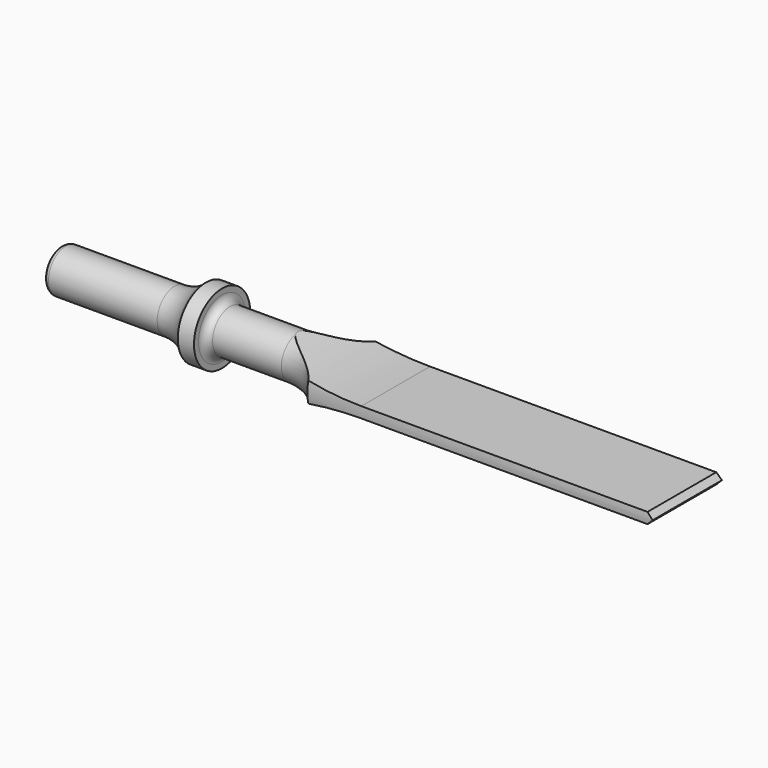
from build123d import *

# Parameters (mm, degrees)
F3_DEPTH = 25.4
F4_DEPTH = 25.4


# Not quite as in the source:
# - ends of sketch curves that miss each other by under 0.0002 mm in the source are joined


with BuildPart() as f1:
    # F0 (on Front) → F1 (revolve)
    with BuildSketch(Plane.XZ):
        with BuildLine():
            Line((0, 4.826), (0, 0))
            Line((0, 0), (184.15, 0))
            Line((184.15, 0), (184.15, 12.7))
            Line((184.15, 12.7), (82.55, 12.7))
            ThreePointArc((82.55, 12.7), (76.9495160289, 8.0259690987), (69.8500007868, 6.350001049))
            Line((69.8500007868, 6.350001049), (49.657, 6.35))
            ThreePointArc((49.657, 6.35), (48.0405538982, 7.0195538982), (47.371, 8.636))
            Line((47.371, 8.636), (47.371, 10.3124))
            Line((47.371, 10.3124), (42.6212, 10.3124))
            ThreePointArc((42.6212, 10.3124), (38.420772371, 7.3825769769), (33.4046742858, 6.35))
            Line((33.4046742858, 6.35), (1.524, 6.35))
            ThreePointArc((1.524, 6.35), (0.4463692655, 5.9036307345), (0, 4.826))
        make_face()
    revolve(axis=Axis((92.075, 0, 0), (1, 0, 0)))

    # F2 (on Front) → F3 (cut)
    with BuildSketch(Plane.XZ):
        with BuildLine():
            Line((189.3032044172, 0), (183.8999837637, 0))
            Line((183.8999837637, 0), (182.3124837637, -1.5875))
            Line((182.3124837637, -1.5875), (98.3069729219, -1.5875))
            ThreePointArc((98.3069729219, -1.5875), (83.7572950904, -2.7862065375), (69.5999860764, -6.35))
            Line((69.5999860764, -6.35), (82.516618073, -56.9406822324))
            Line((82.516618073, -56.9406822324), (124.9158531427, -44.9918061495))
            Line((124.9158531427, -44.9918061495), (189.3032044172, -23.9094942808))
            Line((189.3032044172, -23.9094942808), (189.3032044172, 0))
        make_face()
        with BuildLine():
            Line((182.3124837637, 1.5875), (183.8999837637, 0))
            Line((183.8999837637, 0), (189.3032044172, 0))
            Line((189.3032044172, 0), (189.3032044172, 23.9094942808))
            Line((189.3032044172, 23.9094942808), (183.8999837637, 25.6786675836))
            Line((183.8999837637, 25.6786675836), (124.9158531427, 44.9918061495))
            Line((124.9158531427, 44.9918061495), (82.516618073, 56.9406822324))
            Line((82.516618073, 56.9406822324), (69.5999860764, 6.35))
            ThreePointArc((69.5999860764, 6.35), (83.7572950904, 2.7862065375), (98.3069729219, 1.5875))
            Line((98.3069729219, 1.5875), (182.3124837637, 1.5875))
        make_face()
    extrude(amount=-F3_DEPTH, mode=Mode.SUBTRACT)

    # F2 (on Front) → F4 (cut)
    with BuildSketch(Plane.XZ):
        with BuildLine():
            Line((182.3124837637, 1.5875), (183.8999837637, 0))
            Line((183.8999837637, 0), (189.3032044172, 0))
            Line((189.3032044172, 0), (189.3032044172, 23.9094942808))
            Line((189.3032044172, 23.9094942808), (183.8999837637, 25.6786675836))
            Line((183.8999837637, 25.6786675836), (124.9158531427, 44.9918061495))
            Line((124.9158531427, 44.9918061495), (82.516618073, 56.9406822324))
            Line((82.516618073, 56.9406822324), (69.5999860764, 6.35))
            ThreePointArc((69.5999860764, 6.35), (83.7572950904, 2.7862065375), (98.3069729219, 1.5875))
            Line((98.3069729219, 1.5875), (182.3124837637, 1.5875))
        make_face()
        with BuildLine():
            Line((189.3032044172, 0), (183.8999837637, 0))
            Line((183.8999837637, 0), (182.3124837637, -1.5875))
            Line((182.3124837637, -1.5875), (98.3069729219, -1.5875))
            ThreePointArc((98.3069729219, -1.5875), (83.7572950904, -2.7862065375), (69.5999860764, -6.35))
            Line((69.5999860764, -6.35), (82.516618073, -56.9406822324))
            Line((82.516618073, -56.9406822324), (124.9158531427, -44.9918061495))
            Line((124.9158531427, -44.9918061495), (189.3032044172, -23.9094942808))
            Line((189.3032044172, -23.9094942808), (189.3032044172, 0))
        make_face()
    extrude(amount=F4_DEPTH, mode=Mode.SUBTRACT)


solid = f1.part
